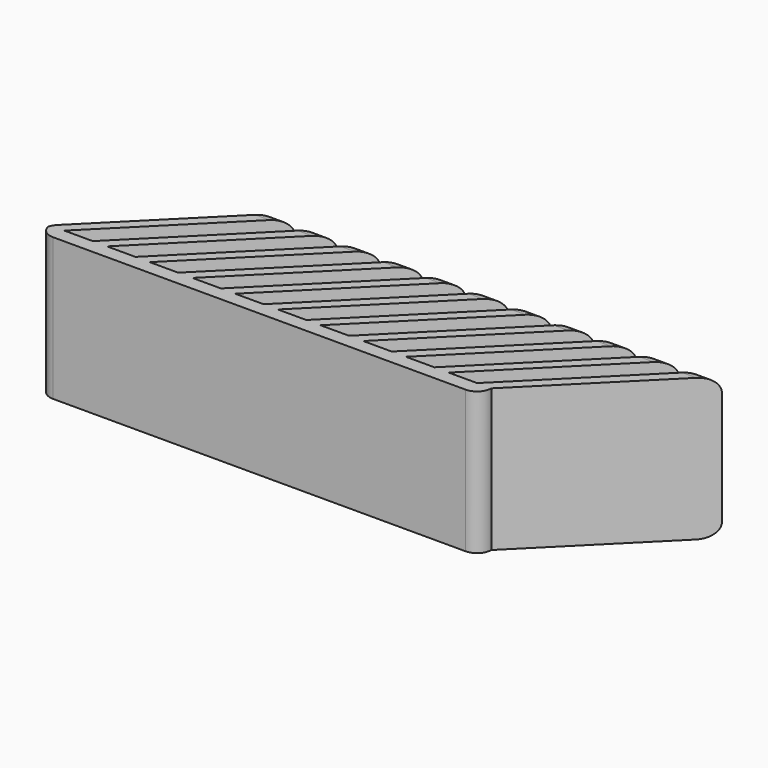
from build123d import *

# Parameters (mm, degrees)
F1_DEPTH     = 25
F2_T1_DEPTH  = 30
F2_T3_DEPTH  = 30
F2_T5_DEPTH  = 30
F2_T7_DEPTH  = 30
F2_T9_DEPTH  = 30
F2_T11_DEPTH = 30
F2_T13_DEPTH = 30
F2_T15_DEPTH = 30
F2_T17_DEPTH = 30
F2_T19_DEPTH = 30
F2_T21_DEPTH = 30
F2_T23_DEPTH = 60.3553390593
F2_T25_DEPTH = 75


# Not quite as in the source:
# - a fillet or chamfer that OpenCascade refuses, or shapes differently, is made with other operations: its cross-section is extruded or revolved along the edge and cut away or added


with BuildPart() as f1:
    # F0 (on Top) → F1 (new body, symmetric)
    with BuildSketch(Plane.XY):
        Polygon((-56.5580020845, 10.0351088219), (-69.7381969311, -3.1450860247), (-101.5580020845, -34.9648911781), (-96.5580020845, -34.9648911781), (-51.5580020845, 10.0351088219), align=None)
        Polygon((-96.5580020845, -34.9648911781), (-101.5580020845, -34.9648911781), (-101.5580020845, -39.9648911781), (53.4419979155, -39.9648911781), (53.4419979155, -34.9648911781), (48.4419979155, -34.9648911781), (38.4419979155, -34.9648911781), (33.4419979155, -34.9648911781), (23.4419979155, -34.9648911781), (18.4419979155, -34.9648911781), (8.4419979155, -34.9648911781), (3.4419979155, -34.9648911781), (-6.5580020845, -34.9648911781), (-11.5580020845, -34.9648911781), (-21.5580020845, -34.9648911781), (-26.5580020845, -34.9648911781), (-36.5580020845, -34.9648911781), (-41.5580020845, -34.9648911781), (-51.5580020845, -34.9648911781), (-56.5580020845, -34.9648911781), (-66.5580020845, -34.9648911781), (-71.5580020845, -34.9648911781), (-81.5580020845, -34.9648911781), (-86.5580020845, -34.9648911781), align=None)
        Polygon((-41.5580020845, 10.0351088219), (-86.5580020845, -34.9648911781), (-81.5580020845, -34.9648911781), (-36.5580020845, 10.0351088219), align=None)
        Polygon((48.4419979155, -34.9648911781), (53.4419979155, -34.9648911781), (98.4419979155, 10.0351088219), (93.4419979155, 10.0351088219), align=None)
        Polygon((-26.5580020845, 10.0351088219), (-71.5580020845, -34.9648911781), (-66.5580020845, -34.9648911781), (-21.5580020845, 10.0351088219), align=None)
        Polygon((33.4419979155, -34.9648911781), (38.4419979155, -34.9648911781), (83.4419979155, 10.0351088219), (78.4419979155, 10.0351088219), align=None)
        Polygon((-11.5580020845, 10.0351088219), (-56.5580020845, -34.9648911781), (-51.5580020845, -34.9648911781), (-6.5580020845, 10.0351088219), align=None)
        Polygon((18.4419979155, -34.9648911781), (23.4419979155, -34.9648911781), (68.4419979155, 10.0351088219), (63.4419979155, 10.0351088219), align=None)
        Polygon((3.4419979155, 10.0351088219), (-41.5580020845, -34.9648911781), (-36.5580020845, -34.9648911781), (8.4419979155, 10.0351088219), align=None)
        Polygon((3.4419979155, -34.9648911781), (8.4419979155, -34.9648911781), (53.4419979155, 10.0351088219), (48.4419979155, 10.0351088219), align=None)
        Polygon((18.4419979155, 10.0351088219), (-26.5580020845, -34.9648911781), (-21.5580020845, -34.9648911781), (23.4419979155, 10.0351088219), align=None)
        Polygon((-11.5580020845, -34.9648911781), (-6.5580020845, -34.9648911781), (38.4419979155, 10.0351088219), (33.4419979155, 10.0351088219), align=None)
    extrude(amount=F1_DEPTH, both=True)

    # F2: fillet of radius 5 on 25 edges, made by hand

    # F2_s2 → F2_t1 (cut)
    with BuildSketch(Plane.YZ.offset(-69.0580020845)):
        with BuildLine():
            ThreePointArc((10.0351088219, -20), (8.5706427278, -23.5355339059), (5.0351088219, -25))
            Line((5.0351088219, -25), (10.0351088219, -25))
            Line((10.0351088219, -25), (10.0351088219, -20))
        make_face()
        with BuildLine():
            ThreePointArc((10.0351088219, 20), (8.5706427278, 23.5355339059), (5.0351088219, 25))
            Line((5.0351088219, 25), (10.0351088219, 25))
            Line((10.0351088219, 25), (10.0351088219, 20))
        make_face()
    extrude(amount=F2_T1_DEPTH, mode=Mode.SUBTRACT)

    # F2_s4 → F2_t3 (cut)
    with BuildSketch(Plane.YZ.offset(-54.0580020845)):
        with BuildLine():
            ThreePointArc((10.0351088219, 20), (8.5706427278, 23.5355339059), (5.0351088219, 25))
            Line((5.0351088219, 25), (10.0351088219, 25))
            Line((10.0351088219, 25), (10.0351088219, 20))
        make_face()
        with BuildLine():
            ThreePointArc((10.0351088219, -20), (8.5706427278, -23.5355339059), (5.0351088219, -25))
            Line((5.0351088219, -25), (10.0351088219, -25))
            Line((10.0351088219, -25), (10.0351088219, -20))
        make_face()
    extrude(amount=F2_T3_DEPTH, mode=Mode.SUBTRACT)

    # F2_s6 → F2_t5 (cut)
    with BuildSketch(Plane.YZ.offset(-39.0580020845)):
        with BuildLine():
            ThreePointArc((10.0351088219, -20), (8.5706427278, -23.5355339059), (5.0351088219, -25))
            Line((5.0351088219, -25), (10.0351088219, -25))
            Line((10.0351088219, -25), (10.0351088219, -20))
        make_face()
        with BuildLine():
            ThreePointArc((10.0351088219, 20), (8.5706427278, 23.5355339059), (5.0351088219, 25))
            Line((5.0351088219, 25), (10.0351088219, 25))
            Line((10.0351088219, 25), (10.0351088219, 20))
        make_face()
    extrude(amount=F2_T5_DEPTH, mode=Mode.SUBTRACT)

    # F2_s8 → F2_t7 (cut)
    with BuildSketch(Plane.YZ.offset(-24.0580020845)):
        with BuildLine():
            ThreePointArc((10.0351088219, 20), (8.5706427278, 23.5355339059), (5.0351088219, 25))
            Line((5.0351088219, 25), (10.0351088219, 25))
            Line((10.0351088219, 25), (10.0351088219, 20))
        make_face()
        with BuildLine():
            ThreePointArc((10.0351088219, -20), (8.5706427278, -23.5355339059), (5.0351088219, -25))
            Line((5.0351088219, -25), (10.0351088219, -25))
            Line((10.0351088219, -25), (10.0351088219, -20))
        make_face()
    extrude(amount=F2_T7_DEPTH, mode=Mode.SUBTRACT)

    # F2_s10 → F2_t9 (cut)
    with BuildSketch(Plane.YZ.offset(-9.0580020845)):
        with BuildLine():
            ThreePointArc((10.0351088219, 20), (8.5706427278, 23.5355339059), (5.0351088219, 25))
            Line((5.0351088219, 25), (10.0351088219, 25))
            Line((10.0351088219, 25), (10.0351088219, 20))
        make_face()
        with BuildLine():
            ThreePointArc((10.0351088219, -20), (8.5706427278, -23.5355339059), (5.0351088219, -25))
            Line((5.0351088219, -25), (10.0351088219, -25))
            Line((10.0351088219, -25), (10.0351088219, -20))
        make_face()
    extrude(amount=F2_T9_DEPTH, mode=Mode.SUBTRACT)

    # F2_s12 → F2_t11 (cut)
    with BuildSketch(Plane.YZ.offset(5.9419979155)):
        with BuildLine():
            ThreePointArc((10.0351088219, -20), (8.5706427278, -23.5355339059), (5.0351088219, -25))
            Line((5.0351088219, -25), (10.0351088219, -25))
            Line((10.0351088219, -25), (10.0351088219, -20))
        make_face()
        with BuildLine():
            ThreePointArc((10.0351088219, 20), (8.5706427278, 23.5355339059), (5.0351088219, 25))
            Line((5.0351088219, 25), (10.0351088219, 25))
            Line((10.0351088219, 25), (10.0351088219, 20))
        make_face()
    extrude(amount=F2_T11_DEPTH, mode=Mode.SUBTRACT)

    # F2_s14 → F2_t13 (cut)
    with BuildSketch(Plane.YZ.offset(20.9419979155)):
        with BuildLine():
            ThreePointArc((10.0351088219, 20), (8.5706427278, 23.5355339059), (5.0351088219, 25))
            Line((5.0351088219, 25), (10.0351088219, 25))
            Line((10.0351088219, 25), (10.0351088219, 20))
        make_face()
        with BuildLine():
            ThreePointArc((10.0351088219, -20), (8.5706427278, -23.5355339059), (5.0351088219, -25))
            Line((5.0351088219, -25), (10.0351088219, -25))
            Line((10.0351088219, -25), (10.0351088219, -20))
        make_face()
    extrude(amount=F2_T13_DEPTH, mode=Mode.SUBTRACT)

    # F2_s16 → F2_t15 (cut)
    with BuildSketch(Plane.YZ.offset(35.9419979155)):
        with BuildLine():
            ThreePointArc((10.0351088219, 20), (8.5706427278, 23.5355339059), (5.0351088219, 25))
            Line((5.0351088219, 25), (10.0351088219, 25))
            Line((10.0351088219, 25), (10.0351088219, 20))
        make_face()
        with BuildLine():
            ThreePointArc((10.0351088219, -20), (8.5706427278, -23.5355339059), (5.0351088219, -25))
            Line((5.0351088219, -25), (10.0351088219, -25))
            Line((10.0351088219, -25), (10.0351088219, -20))
        make_face()
    extrude(amount=F2_T15_DEPTH, mode=Mode.SUBTRACT)

    # F2_s18 → F2_t17 (cut)
    with BuildSketch(Plane.YZ.offset(50.9419979155)):
        with BuildLine():
            ThreePointArc((10.0351088219, 20), (8.5706427278, 23.5355339059), (5.0351088219, 25))
            Line((5.0351088219, 25), (10.0351088219, 25))
            Line((10.0351088219, 25), (10.0351088219, 20))
        make_face()
        with BuildLine():
            ThreePointArc((10.0351088219, -20), (8.5706427278, -23.5355339059), (5.0351088219, -25))
            Line((5.0351088219, -25), (10.0351088219, -25))
            Line((10.0351088219, -25), (10.0351088219, -20))
        make_face()
    extrude(amount=F2_T17_DEPTH, mode=Mode.SUBTRACT)

    # F2_s20 → F2_t19 (cut)
    with BuildSketch(Plane.YZ.offset(65.9419979155)):
        with BuildLine():
            ThreePointArc((10.0351088219, 20), (8.5706427278, 23.5355339059), (5.0351088219, 25))
            Line((5.0351088219, 25), (10.0351088219, 25))
            Line((10.0351088219, 25), (10.0351088219, 20))
        make_face()
        with BuildLine():
            ThreePointArc((10.0351088219, -20), (8.5706427278, -23.5355339059), (5.0351088219, -25))
            Line((5.0351088219, -25), (10.0351088219, -25))
            Line((10.0351088219, -25), (10.0351088219, -20))
        make_face()
    extrude(amount=F2_T19_DEPTH, mode=Mode.SUBTRACT)

    # F2_s22 → F2_t21 (cut)
    with BuildSketch(Plane.YZ.offset(80.9419979155)):
        with BuildLine():
            ThreePointArc((10.0351088219, 20), (8.5706427278, 23.5355339059), (5.0351088219, 25))
            Line((5.0351088219, 25), (10.0351088219, 25))
            Line((10.0351088219, 25), (10.0351088219, 20))
        make_face()
        with BuildLine():
            ThreePointArc((10.0351088219, -20), (8.5706427278, -23.5355339059), (5.0351088219, -25))
            Line((5.0351088219, -25), (10.0351088219, -25))
            Line((10.0351088219, -25), (10.0351088219, -20))
        make_face()
    extrude(amount=F2_T21_DEPTH, mode=Mode.SUBTRACT)

    # F2_s24 → F2_t23 (cut)
    with BuildSketch(Plane.XY.offset(-30.1776695297)):
        with BuildLine():
            ThreePointArc((-100.0935359904, -33.5004250841), (-101.1773997471, -35.1225418282), (-101.5580020845, -37.03595899))
            Line((-101.5580020845, -37.03595899), (-101.5580020845, -34.9648911781))
            Line((-101.5580020845, -34.9648911781), (-100.0935359904, -33.5004250841))
        make_face()
    extrude(amount=F2_T23_DEPTH, mode=Mode.SUBTRACT)

    # F2_s26 → F2_t25 (cut)
    with BuildSketch(Plane.XY.offset(-37.5)):
        with BuildLine():
            ThreePointArc((-96.5580020845, -39.9648911781), (-100.0935359904, -38.5004250841), (-101.5580020845, -34.9648911781))
            Line((-101.5580020845, -34.9648911781), (-101.5580020845, -39.9648911781))
            Line((-101.5580020845, -39.9648911781), (-96.5580020845, -39.9648911781))
        make_face()
        with BuildLine():
            ThreePointArc((53.4419979155, -34.9648911781), (51.9775318214, -38.5004250841), (48.4419979155, -39.9648911781))
            Line((48.4419979155, -39.9648911781), (53.4419979155, -39.9648911781))
            Line((53.4419979155, -39.9648911781), (53.4419979155, -34.9648911781))
        make_face()
    extrude(amount=F2_T25_DEPTH, mode=Mode.SUBTRACT)


solid = f1.part
